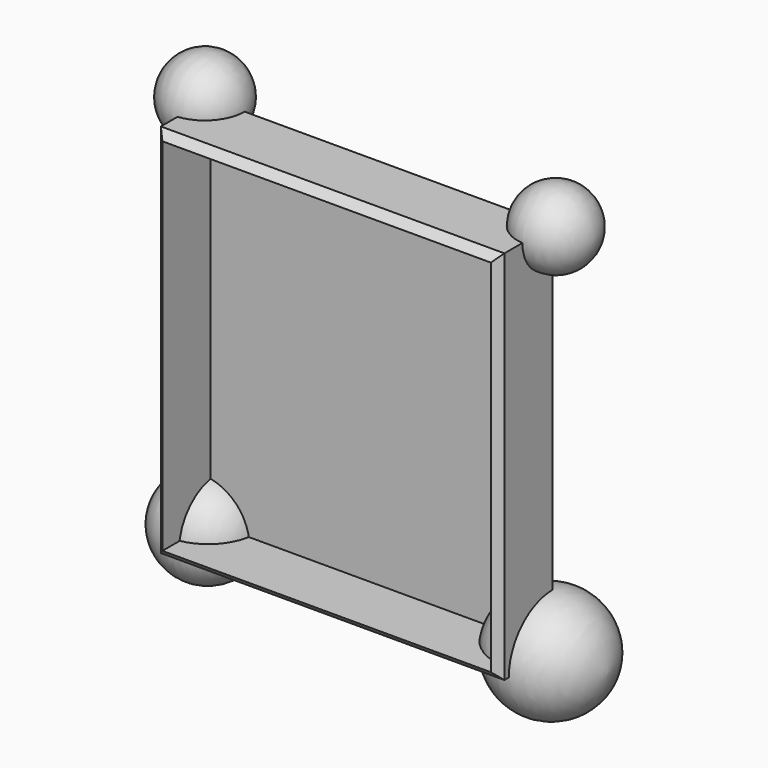
from build123d import *

# Parameters (mm, degrees)
F5_DEPTH    = 25.4
F6_T        = -2.54
F7_T1_DEPTH = 141.7753282894
F7_T3_DEPTH = 152.591246735


# Not quite as in the source:
# - a fillet or chamfer that OpenCascade refuses, or shapes differently, is made with other operations: its cross-section is extruded or revolved along the edge and cut away or added


with BuildPart() as f1:
    # F0 (on Front) → F1 (revolve)
    with BuildSketch(Plane.XZ):
        with BuildLine():
            Line((-75.7113620639, 50.3355823457), (-63.7607946992, 50.3355823457))
            ThreePointArc((-63.7607946992, 50.3355823457), (-77.1189443767, 63.7302291931), (-90.4770940542, 50.3355823457))
            Line((-90.4770940542, 50.3355823457), (-75.7113620639, 50.3355823457))
        make_face()
    revolve(axis=Axis((-77.1189443767, 0, 50.3355823457), (-1, 0, 0)))


with BuildPart() as f2:
    # F0 (on Front) → F2 (revolve)
    with BuildSketch(Plane.XZ):
        with BuildLine():
            Line((27.9321912676, 50.3355823457), (39.9356670678, 50.3355823457))
            Line((39.9356670678, 50.3355823457), (53.9888329804, 50.3355823457))
            ThreePointArc((53.9888329804, 50.3355823457), (40.960512124, 63.1556217242), (27.9321912676, 50.3355823457))
        make_face()
    revolve(axis=Axis((40.960512124, 0, 50.3355823457), (1, 0, 0)))


with BuildPart() as f3:
    # F0 (on Front) → F3 (revolve)
    with BuildSketch(Plane.XZ):
        with BuildLine():
            ThreePointArc((-92.759013176, -76.1273652315), (-76.3068143278, -92.2774497957), (-59.8546154797, -76.1273652315))
            Line((-59.8546154797, -76.1273652315), (-75.7113620639, -76.1273652315))
            Line((-75.7113620639, -76.1273652315), (-92.759013176, -76.1273652315))
        make_face()
    revolve(axis=Axis((-76.3068143278, 0, -76.1273652315), (-1, 0, 0)))


with BuildPart() as f4:
    # F0 (on Front) → F4 (revolve)
    with BuildSketch(Plane.XZ):
        with BuildLine():
            Line((58.6881376803, -76.1273652315), (39.9356670678, -76.1273652315))
            Line((39.9356670678, -76.1273652315), (19.7396241128, -76.1273652315))
            ThreePointArc((19.7396241128, -76.1273652315), (39.2138808966, -94.6447347989), (58.6881376803, -76.1273652315))
        make_face()
    revolve(axis=Axis((39.2138808966, 0, -76.1273652315), (1, 0, 0)))


with BuildPart() as f5:
    # F0 (on Front) → F5 (new body)
    with BuildSketch(Plane.XZ):
        Polygon((39.9356670678, -76.1273652315), (39.9356670678, 50.3355823457), (27.9321912676, 50.3355823457), (-63.7607946992, 50.3355823457), (-75.7113620639, 50.3355823457), (-75.7113620639, -76.1273652315), (-59.8546154797, -76.1273652315), (19.7396241128, -76.1273652315), align=None)
    extrude(amount=F5_DEPTH)

    # F6
    f6_openings = [f5.faces().sort_by_distance(p)[0] for p in [
        (-17.887847, -25.4, -12.895891),
    ]]
    offset(amount=F6_T, openings=f6_openings)

    # F7: chamfer of 5.08 on 4 edges, made by hand

    # F7_s2 → F7_t1 (cut)
    with BuildSketch(Plane.YZ.offset(-88.7755116428)):
        Polygon((-20.32, -76.1273652315), (-25.4, -71.0473652315), (-25.4, -76.1273652315), align=None)
        Polygon((-20.32, 50.3355823457), (-25.4, 45.2555823457), (-25.4, 50.3355823457), align=None)
    extrude(amount=F7_T1_DEPTH, mode=Mode.SUBTRACT)

    # F7_s4 → F7_t3 (cut)
    with BuildSketch(Plane.XY.offset(-89.1915148104)):
        Polygon((39.9356670678, -20.32), (34.8556670678, -25.4), (39.9356670678, -25.4), align=None)
        Polygon((-75.7113620639, -20.32), (-70.6313620639, -25.4), (-75.7113620639, -25.4), align=None)
    extrude(amount=F7_T3_DEPTH, mode=Mode.SUBTRACT)


solid = Compound([f1.part, f2.part, f3.part, f4.part, f5.part])
